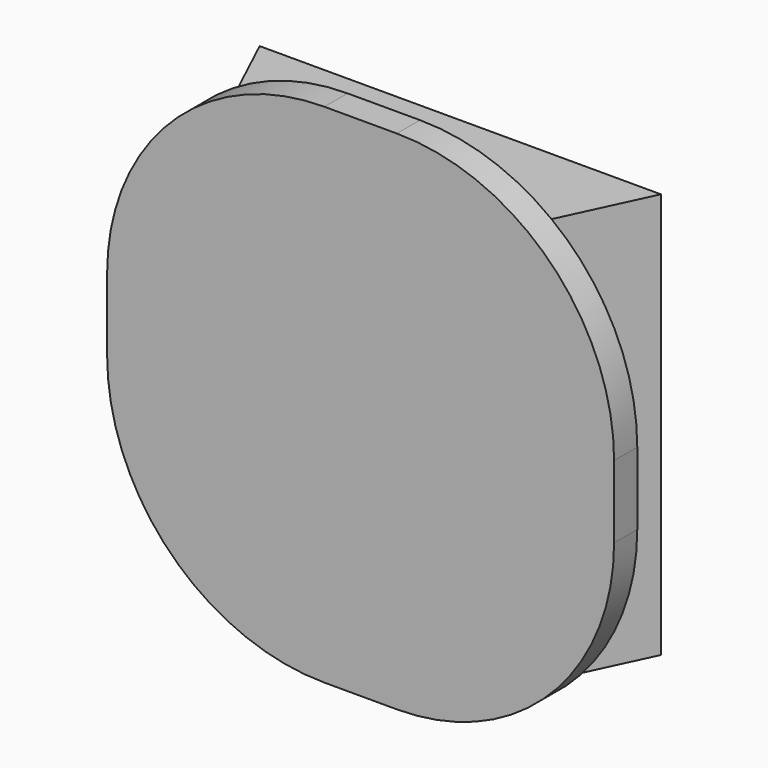
from build123d import *

# Parameters (mm, degrees)
F1_DEPTH     = 6
F3_DEPTH     = 15
F5_DEPTH     = 5.0000008951
F6_R         = 5
F10_DEPTH    = 5
F11_W        = 35
F11_H        = 35
F12_DEPTH    = 2
F15_W        = 27.7
F15_H        = 28
F13_W        = 21.5
F13_H        = 28
F17_T        = 2.5
F17_T3_DEPTH = 26.5
F17_T5_DEPTH = 33
F19_R        = 2.5
F20_DEPTH    = 54.5
F21_R        = 15
F22_R        = 3
F23_R        = 0.5
F24_R        = 2
F25_R        = 6
F28_DEPTH    = 0.3


# Not quite as in the source:
# - ends of sketch curves that miss each other by under 0.0002 mm in the source are joined
# - a shell that OpenCascade refuses in one call is made with other operations: the cavity is built on its own and cut out


with BuildPart() as f1:
    # F0 (on Top) → F1 (new body)
    with BuildSketch(Plane.XY):
        Polygon((11.0000005256, -18.05), (11.0000005256, -20.55), (-11.0000005256, -20.55), (-10.9999994744, 20.55), (11.0000005256, 20.55), (11.0000005256, 18.05), (15.8927322497, 21.8000001848), (16.1137396651, 25.5500003695), (11.4420153564, 25.5500003695), (-15.9999997161, 25.5500003695), (-16.000001023, -25.5500003695), (11.4420153564, -25.5500003695), (16.1137396651, -25.5500003695), (15.8927322497, -21.8000001848), align=None)
    extrude(amount=F1_DEPTH)

    # F2 (on face) → F3 (join)
    with BuildSketch(Plane(origin=(0, 0, 0), x_dir=(1, 0, 0), z_dir=(0, 0, -1))):
        Polygon((-10.9999994744, -25.5500003695), (-15.9999997161, -25.5500003695), (-15.9999997161, -40.5500003695), (-10.9999994744, -40.5500003695), (4.0000002839, -40.5500003695), (4.0000002839, -36.5500003695), (-10.9999994744, -36.5500003695), align=None)
    extrude(amount=-F3_DEPTH)

    # F4 (on face) → F5 (cut, through all)
    with BuildSketch(Plane.YZ.offset(-10.9999994744)):
        Polygon((25.5500003695, 15), (25.5500003695, 6), (29.5500003695, 6), (36.5500003695, 15), align=None)
    extrude(amount=-F5_DEPTH, mode=Mode.SUBTRACT)

    # F6
    f6_edges = [f1.edges().sort_by_distance(p)[0] for p in [
        (4, 38.55, 15),
    ]]
    fillet(f6_edges, radius=F6_R)


with BuildPart() as f10:
    # F9 (on offset) → F10 (new body)
    with BuildSketch(Plane(origin=(0, 65.5500003695, 0), x_dir=(-1, 0, 0), z_dir=(0, 1, 0))):
        with BuildLine():
            Line((15.9999997161, 0), (15.9999997161, 15))
            Line((15.9999997161, 15), (0.9999997161, 15))
            ThreePointArc((0.9999997161, 15), (-2.5355341898, 13.5355339059), (-4.0000002839, 10))
            Line((-4.0000002839, 10), (-4.0000002839, 0))
            Line((-4.0000002839, 0), (15.9999997161, 0))
        make_face()
    extrude(amount=F10_DEPTH)


with BuildPart() as f12:
    # F11 (on offset) → F12 (new body)
    with BuildSketch(Plane(origin=(0, 88.5500003695, 0), x_dir=(-1, 0, 0), z_dir=(0, 1, 0))):
        with Locations((5.9999997161, 7.5)):
            Rectangle(F11_W, F11_H)
    extrude(amount=F12_DEPTH)

    # F15 (on offset) → F16 section 0
    with BuildSketch(Plane(origin=(0, 97.1500003695, 0), x_dir=(-1, 0, 0), z_dir=(0, 1, 0))):
        with Locations((5.9999997161, 7.5)):
            Rectangle(F15_W, F15_H)
    # F13 (on face) → F16 section 1
    with BuildSketch(Plane(origin=(0, 90.5500003695, 0), x_dir=(-1, 0, 0), z_dir=(0, 1, 0))):
        with Locations((5.9999997161, 7.5)):
            Rectangle(F13_W, F13_H)
    loft()

    # F17: shell of thickness 2.5, made by hand


with BuildPart() as f17_core1:
    # F17_t2: copy of F12
    add(f12.part)

    # the walls: a layer under each face that stays
    f17_faces = [f17_core1.faces().sort_by_distance(p)[0] for p in [
        (-5.9999997161, 89.5500003695, -10),
        (11.5000002839, 89.5500003695, 7.5),
        (-23.4999997161, 89.5500003695, 7.5),
        (-5.9999997161, 88.5500003695, 7.5),
        (5.6666669506, 90.5500003695, -4.1666666667),
        (-5.9999997161, 89.5500003695, 25),
        (-5.9999997161, 93.8500003695, -6.5),
        (-18.2999997161, 93.8500003695, 7.5),
        (-5.9999997161, 93.8500003695, 21.5),
        (6.3000002839, 93.8500003695, 7.5),
    ]]
    thicken(f17_faces, amount=-F17_T, mode=Mode.SUBTRACT)

    # F17_s4 → F17_t3 (cut)
    with BuildSketch(Plane.YZ.offset(-19.2499997161)):
        Polygon((90.5750003695, -6.525), (88.0500003695, -6.5), (88.0500003695, -4), (90.5500003695, -4), align=None)
        Polygon((90.5750003695, 21.525), (88.0500003695, 21.5), (88.0500003695, 19), (90.5500003695, 19), align=None)
    extrude(amount=F17_T3_DEPTH, mode=Mode.SUBTRACT)

    # F17_s6 → F17_t5 (cut)
    with BuildSketch(Plane.XY.offset(-9)):
        Polygon((-16.7726279476, 90.5643719578), (-16.7499997161, 88.0500003695), (-12.8137208564, 88.0500003695), (-14.4871765615, 91.6128415482), align=None)
        Polygon((4.7726285154, 90.5643719578), (4.7500002839, 88.0500003695), (0.8137214242, 88.0500003695), (2.4871771293, 91.6128415482), align=None)
    extrude(amount=F17_T5_DEPTH, mode=Mode.SUBTRACT)


with BuildPart() as f12_1:
    add(f12.part)

    # what is left inside the walls is the cavity
    f17_cavity = [f17_core1.part.solids().sort_by_distance(p)[0] for p in [
        (-2.215544, 97.125, 11.243908),
    ]]
    add(f17_cavity, mode=Mode.SUBTRACT)


with BuildPart() as f20_tool:
    # F19 (on face) → F20 (new body, through all)
    with BuildSketch(Plane(origin=(0, 91.0500003695, 0), x_dir=(-1, 0, 0), z_dir=(0, 1, 0))):
        with Locations((5.9999997161, 7.5)):
            Circle(F19_R)
    extrude(amount=-F20_DEPTH)


with BuildPart() as f1_1:
    add(f1.part)

    # F20: cut by f20_tool
    add(f20_tool.part, mode=Mode.SUBTRACT)

    # F22
    f22_edges = [f1_1.edges().sort_by_distance(p)[0] for p in [
        (-16.000001, -25.55, 3),
        (-10.999999, 25.55, 3),
    ]]
    fillet(f22_edges, radius=F22_R)

    # F23
    f23_edges = [f1_1.edges().sort_by_distance(p)[0] for p in [
        (11.000001, -18.05, 3),
        (11.000001, 18.05, 3),
        (-10.999999, 20.55, 3),
        (-11.000001, -20.55, 3),
    ]]
    fillet(f23_edges, radius=F23_R)

    # F24
    f24_edges = [f1_1.edges().sort_by_distance(p)[0] for p in [
        (-16, 40.55, 7.5),
        (-10.999999, 36.55, 7.5),
    ]]
    fillet(f24_edges, radius=F24_R)

    # F25
    f25_edges = [f1_1.edges().sort_by_distance(p)[0] for p in [
        (-13.5, 29.55, 6),
    ]]
    fillet(f25_edges, radius=F25_R)


with BuildPart() as f12_2:
    add(f12_1.part)

    # F20: cut by f20_tool
    add(f20_tool.part, mode=Mode.SUBTRACT)

    # F21
    f21_edges = [f12_2.edges().sort_by_distance(p)[0] for p in [
        (11.5, 89.55, 25),
        (-23.5, 89.55, 25),
        (-23.5, 89.55, -10),
        (11.5, 89.55, -10),
    ]]
    fillet(f21_edges, radius=F21_R)

    # F27 (on face) → F28 (join)
    with BuildSketch(Plane.XZ.offset(-88.5500003695)):
        with BuildLine():
            ThreePointArc((11.5000002839, 10), (7.1066020017, 20.6066017178), (-3.4999997161, 25))
            Line((-3.4999997161, 25), (-8.4999997161, 25))
            ThreePointArc((-8.4999997161, 25), (-19.1066014339, 20.6066017178), (-23.4999997161, 10))
            Line((-23.4999997161, 10), (-23.4999997161, 5))
            ThreePointArc((-23.4999997161, 5), (-19.1066014339, -5.6066017178), (-8.4999997161, -10))
            Line((-8.4999997161, -10), (-3.4999997161, -10))
            ThreePointArc((-3.4999997161, -10), (7.1066020017, -5.6066017178), (11.5000002839, 5))
            Line((11.5000002839, 5), (11.5000002839, 10))
        make_face()
    extrude(amount=-F28_DEPTH)


solid = f12_2.part
